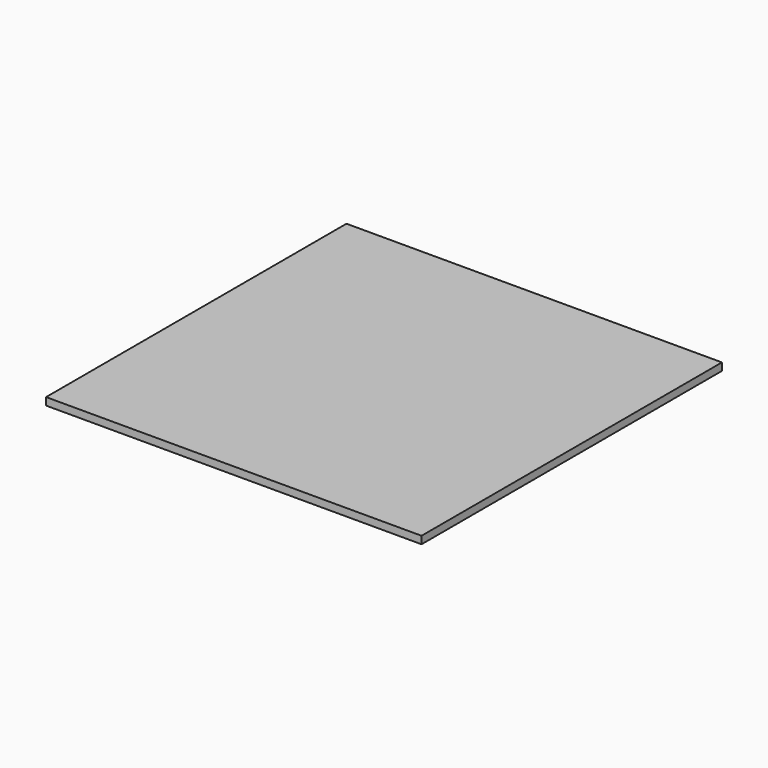
from build123d import *

# Parameters (mm, degrees)
F0_W     = 150
F0_H     = 103
F0_H_2   = 12
F0_H_3   = 25
F0_H_4   = 10
F1_DEPTH = 3


with BuildPart() as f1:
    # F0 (on Top) → F1 (new body)
    with BuildSketch(Plane.XY):
        with Locations((0, 23.5)):
            Rectangle(F0_W, F0_H)
        with Locations((0, -34)):
            Rectangle(F0_W, F0_H_2)
        with Locations((0, -52.5)):
            Rectangle(F0_W, F0_H_3)
        with Locations((0, -70)):
            Rectangle(F0_W, F0_H_4)
    extrude(amount=F1_DEPTH)


solid = f1.part
